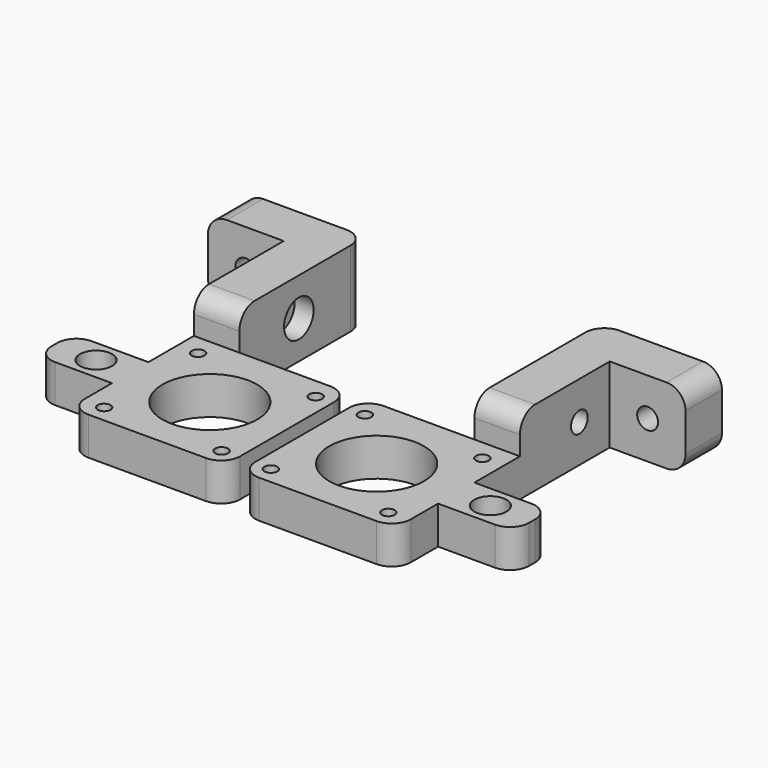
from build123d import *

# Parameters (mm, degrees)
F1_DEPTH             = 20
F2_START             = 10
F0_R                 = 12.5
F0_W                 = 20
F0_H                 = 12
F0_R_2               = 4.25
F2_DEPTH             = 10
F6_D                 = 3.4
F6_CBORE_D           = 6.5
F6_CBORE_DEPTH       = 3
F7_D                 = 5.5
F7_DEPTH             = 30
F7_CBORE_D           = 9.75
F7_CBORE_DEPTH       = 5
F7_TIP               = 1.6523667023
F7_ON_F5_D           = 5.5
F7_ON_F5_DEPTH       = 30
F7_ON_F5_CBORE_D     = 9.75
F7_ON_F5_CBORE_DEPTH = 5
F7_ON_F5_TIP         = 1.6523667023
F8_R                 = 5
F9_ANGLE             = 180


# Not quite as in the source:
# - a feature names something its author has since deleted; it is built from what else it names


with BuildPart() as f1:
    # F0 (on Top) → F1 (new body)
    with BuildSketch(Plane.XY):
        Polygon((43, -56.6), (43, -27), (31, -27), (31, -68.6), (63, -68.6), (63, -56.6), align=None)
    extrude(amount=F1_DEPTH)

    # F0 (on Top) → F2 (join)
    with BuildSketch(Plane.XY.offset(F2_START)):
        Polygon((43, -12), (43, 0), (43, 14), (2, 14), (2, -27), (31, -27), (43, -27), align=None)
        with Locations((22, -6)):
            Circle(F0_R, mode=Mode.SUBTRACT)
        with Locations((53, -6)):
            Rectangle(F0_W, F0_H)
        with Locations((52, -6)):
            Circle(F0_R_2, mode=Mode.SUBTRACT)
    extrude(amount=F2_DEPTH)

    # F6 (through all)
    with Locations(Plane.XY.offset(20)):
        with Locations((6.5, 9.5), (37.5, 9.5), (37.5, -21.5), (6.5, -21.5)):
            CounterBoreHole(F6_D / 2, F6_CBORE_D / 2, F6_CBORE_DEPTH)

    # F7
    with Locations(Plane(origin=(31, 0, 0), x_dir=(0, -1, 0), z_dir=(-1, 0, 0))):
        with Locations((46.6, 10)):
            CounterBoreHole(F7_D / 2, F7_CBORE_D / 2, F7_CBORE_DEPTH, depth=F7_DEPTH)
            with Locations((0, 0, -(F7_DEPTH + F7_TIP / 2))):  # 118° drill point
                Cone(0, F7_D / 2, F7_TIP, mode=Mode.SUBTRACT)

    # F7 on F5
    with Locations(Plane.XZ.offset(68.6)):
        with Locations((53, 10)):
            CounterBoreHole(F7_ON_F5_D / 2, F7_ON_F5_CBORE_D / 2, F7_ON_F5_CBORE_DEPTH, depth=F7_ON_F5_DEPTH)
            with Locations((0, 0, -(F7_ON_F5_DEPTH + F7_ON_F5_TIP / 2))):  # 118° drill point
                Cone(0, F7_ON_F5_D / 2, F7_ON_F5_TIP, mode=Mode.SUBTRACT)

    # F8
    f8_edges = [f1.edges().sort_by_distance(p)[0] for p in [
        (2, 14, 15),
        (43, 14, 15),
        (2, -27, 15),
        (63, 0, 15),
        (63, -12, 15),
        (37, -27, 0),
        (63, -62.6, 0),
        (63, -62.6, 20),
        (31, -68.6, 10),
    ]]
    fillet(f8_edges, radius=F8_R)


with BuildPart() as f1_1:
    # F9: moved
    add(f1.part.rotate(Axis((22.5, 14, 20), (-1, 0, 0)), F9_ANGLE))


with BuildPart() as f10_1:
    # F10: instance of F1
    add(f1_1.part.mirror(Plane.YZ))


solid = Compound([f1_1.part, f10_1.part])
